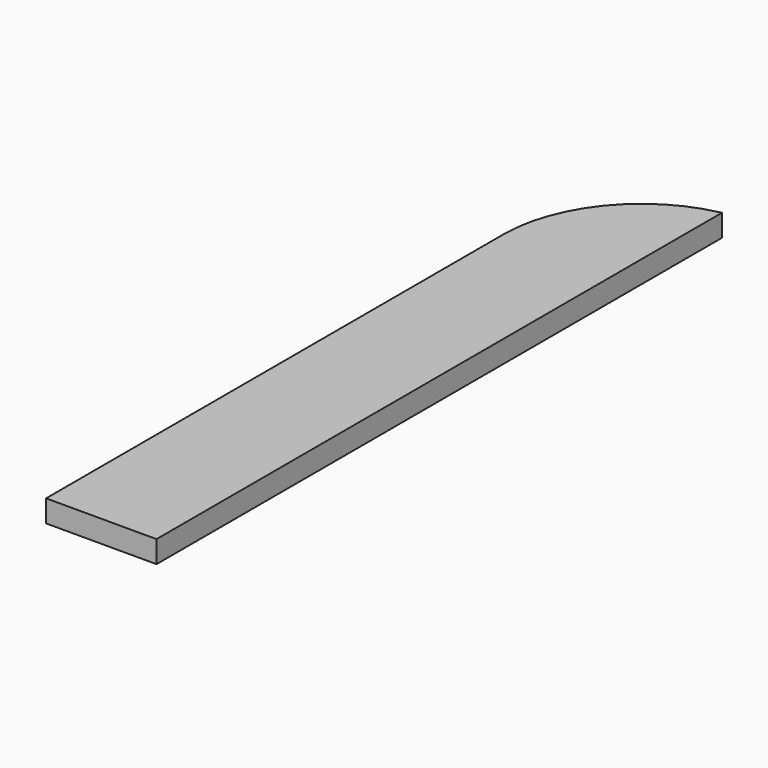
from build123d import *

# Parameters (mm, degrees)
F0_W        = 508
F0_H        = 3251.2
F1_DEPTH    = 101.6
F2_T1_DEPTH = 3212.4519733346


# Not quite as in the source:
# - a fillet or chamfer that OpenCascade refuses, or shapes differently, is made with other operations: its cross-section is extruded or revolved along the edge and cut away or added


with BuildPart() as f1:
    # F0 (on Top) → F1 (new body)
    with BuildSketch(Plane.XY):
        Rectangle(F0_W, F0_H)
    extrude(amount=F1_DEPTH)

    # F2: fillet of radius 635 on 1 edges, made by hand

    # F2_s2 → F2_t1 (cut)
    with BuildSketch(Plane.XY.offset(-1555.4259866673)):
        with BuildLine():
            ThreePointArc((254, 1625.6), (-110.8688849683, 1405.0388681745), (-254, 1003.4296053331))
            Line((-254, 1003.4296053331), (-254, 1625.6))
            Line((-254, 1625.6), (254, 1625.6))
        make_face()
    extrude(amount=F2_T1_DEPTH, mode=Mode.SUBTRACT)


solid = f1.part
